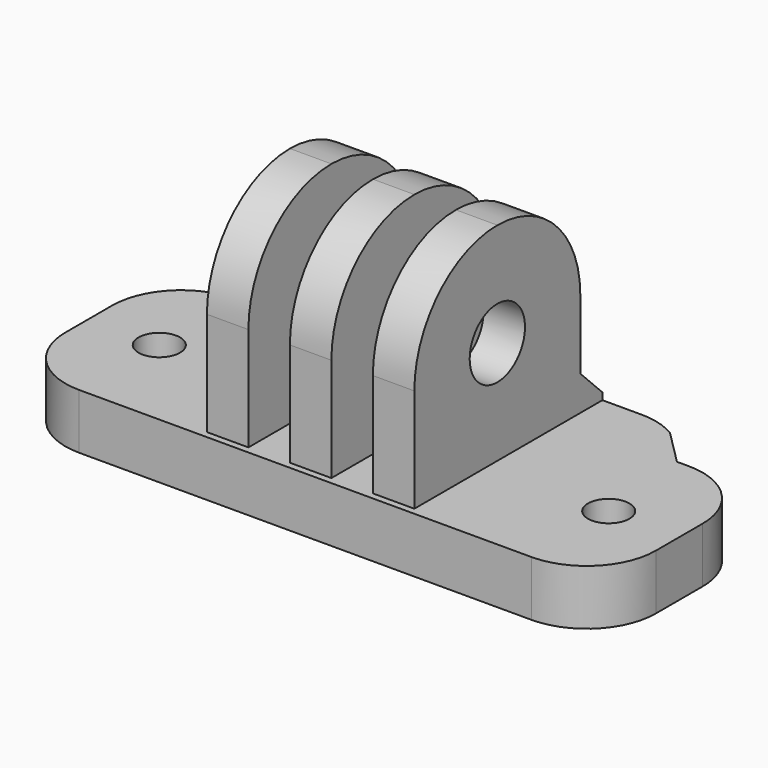
from build123d import *

# Parameters (mm, degrees)
F0_R         = 1.5
F0_W         = 3
F0_H         = 13.7437733207
F0_H_2       = 1.2562266793
F1_DEPTH     = 4
F2_DEPTH     = 19
F3_R         = 7.49999
F4_R         = 2.5
F5_DEPTH     = 28.851
F6_T1_DEPTH  = 4
F6_T6_DEPTH  = 3
F6_T11_DEPTH = 9.4292074699
F6_T18_DEPTH = 9.4292074699
F6_T25_DEPTH = 3
F6_T30_DEPTH = 9.4292074699
F6_T37_DEPTH = 9.4292074699
F6_T44_DEPTH = 3
F7_T1_DEPTH  = 17.2196709514
F7_T3_DEPTH  = 29


# Not quite as in the source:
# - a fillet or chamfer that OpenCascade refuses, or shapes differently, is made with other operations: its cross-section is extruded or revolved along the edge and cut away or added
# - a fillet or chamfer is up to 0.001 mm smaller than in the source, because OpenCascade refuses the exact size


with BuildPart() as f1:
    # F0 (on Top) → F1 (new body)
    with BuildSketch(Plane.XY):
        Polygon((-12.9930239742, 7.1134486855), (-21.35, 7.1134486855), (-21.35, -7.1134486855), (21.35, -7.1134486855), (21.35, 7.1134486855), (12.9930239742, 7.1134486855), (7.5, 7.1134486855), (7.5, -6.6303246352), (4.5, -6.6303246352), (4.5, 7.1134486855), (1.5, 7.1134486855), (1.5, -6.6303246352), (-1.5, -6.6303246352), (-1.5, 7.1134486855), (-4.5, 7.1134486855), (-4.5, -6.6303246352), (-7.5, -6.6303246352), (-7.5, 7.1134486855), align=None)
        with Locations((-16.25, 0)):
            Circle(F0_R, mode=Mode.SUBTRACT)
        with Locations((16.25, 0)):
            Circle(F0_R, mode=Mode.SUBTRACT)
        Polygon((-12.9930239742, 10.3696753648), (-12.9930239742, 7.1134486855), (-7.5, 7.1134486855), (-7.5, 8.3696753648), (-4.5, 8.3696753648), (-1.5, 8.3696753648), (1.5, 8.3696753648), (4.5, 8.3696753648), (7.5, 8.3696753648), (7.5, 7.1134486855), (12.9930239742, 7.1134486855), (12.9930239742, 10.3696753648), align=None)
        with Locations((-6, 0.2415620252)):
            Rectangle(F0_W, F0_H)
        with Locations((-6, 7.7415620252)):
            Rectangle(F0_W, F0_H_2)
        with Locations((-3, 7.7415620252)):
            Rectangle(F0_W, F0_H_2)
        Polygon((-1.5, 8.3696753648), (-1.5, 7.1134486855), (0, 7.1134486855), (1.5, 7.1134486855), (1.5, 8.3696753648), align=None)
        Polygon((0, 7.1134486855), (-1.5, 7.1134486855), (-1.5, -6.6303246352), (1.5, -6.6303246352), (1.5, 7.1134486855), align=None)
        with Locations((3, 7.7415620252)):
            Rectangle(F0_W, F0_H_2)
        with Locations((6, 0.2415620252)):
            Rectangle(F0_W, F0_H)
        with Locations((6, 7.7415620252)):
            Rectangle(F0_W, F0_H_2)
    extrude(amount=F1_DEPTH)

    # F0 (on Top) → F2 (join)
    with BuildSketch(Plane.XY):
        with Locations((-6, 0.2415620252)):
            Rectangle(F0_W, F0_H)
        with Locations((-6, 7.7415620252)):
            Rectangle(F0_W, F0_H_2)
        Polygon((-1.5, 8.3696753648), (-1.5, 7.1134486855), (0, 7.1134486855), (1.5, 7.1134486855), (1.5, 8.3696753648), align=None)
        Polygon((0, 7.1134486855), (-1.5, 7.1134486855), (-1.5, -6.6303246352), (1.5, -6.6303246352), (1.5, 7.1134486855), align=None)
        with Locations((6, 0.2415620252)):
            Rectangle(F0_W, F0_H)
        with Locations((6, 7.7415620252)):
            Rectangle(F0_W, F0_H_2)
    extrude(amount=F2_DEPTH)

    # F3 (radius 7.5 in the source; OpenCascade refuses exactly that, so slightly less here)
    f3_edges = [f1.edges().sort_by_distance(p)[0] for p in [
        (-6, -6.630325, 19),
        (0, -6.630325, 19),
        (6, -6.630325, 19),
        (6, 8.369675, 19),
        (0, 8.369675, 19),
        (-6, 8.369675, 19),
    ]]
    fillet(f3_edges, radius=F3_R)

    # F4 (on face) → F5 (cut, through all)
    with BuildSketch(Plane(origin=(-7.5, 0, 0), x_dir=(0, -1, 0), z_dir=(-1, 0, 0))):
        with Locations((-0.8696753648, 11.5)):
            Circle(F4_R)
    extrude(amount=-F5_DEPTH, mode=Mode.SUBTRACT)

    # F6: chamfer of 2.5 on 5 edges, made by hand

    # F6_s2 → F6_t1 (join)
    with BuildSketch(Plane.XY):
        Polygon((12.9930239742, 9.6134486855), (15.4930239742, 7.1134486855), (12.9930239742, 7.1134486855), align=None)
        Polygon((-15.4930239742, 7.1134486855), (-12.9930239742, 9.6134486855), (-12.9930239742, 7.1134486855), align=None)
    extrude(amount=F6_T1_DEPTH)


with BuildPart() as f6_tool4:
    # F6_s5 → F6_t6 (new body)
    with BuildSketch(Plane.YZ.offset(-7.5)):
        Polygon((8.3696753648, 6.5), (10.8696753648, 4), (8.3696753648, 4), align=None)
    extrude(amount=F6_T6_DEPTH)

    split(bisect_by=Plane.XZ.offset(-10.3696753648), keep=Keep.TOP)


with BuildPart() as f1_1:
    add(f1.part)

    # F6_t3: union F6_tool4
    add(f6_tool4.part)


with BuildPart() as f6_tool9:
    # F6_s10 → F6_t11 (new body)
    with BuildSketch(Plane.YZ.offset(-7.5)):
        Polygon((8.3696753648, 6.5), (10.8696753648, 4), (8.3696753648, 4), align=None)
    extrude(amount=F6_T11_DEPTH)

    split(bisect_by=Plane.XZ.offset(-10.3696753648), keep=Keep.TOP)

    split(bisect_by=Plane.YZ.offset(-1.5), keep=Keep.TOP)

    split(bisect_by=Plane.YZ.offset(1.5), keep=Keep.BOTTOM)


with BuildPart() as f1_2:
    add(f1_1.part)

    # F6_t8: union F6_tool9
    add(f6_tool9.part)


with BuildPart() as f6_tool16:
    # F6_s17 → F6_t18 (new body)
    with BuildSketch(Plane.YZ.offset(-7.9292074699)):
        Polygon((10.8696753648, 4), (8.3696753648, 6.5), (8.3696753648, 4), align=None)
    extrude(amount=F6_T18_DEPTH)

    split(bisect_by=Plane.YZ.offset(-7.5), keep=Keep.TOP)

    split(bisect_by=Plane.YZ.offset(-4.5), keep=Keep.BOTTOM)

    split(bisect_by=Plane.XZ.offset(-10.3696753648), keep=Keep.TOP)


with BuildPart() as f1_3:
    add(f1_2.part)

    # F6_t15: union F6_tool16
    add(f6_tool16.part)


with BuildPart() as f6_tool23:
    # F6_s24 → F6_t25 (new body)
    with BuildSketch(Plane.YZ.offset(-1.5)):
        Polygon((10.8696753648, 4), (8.3696753648, 6.5), (8.3696753648, 4), align=None)
    extrude(amount=F6_T25_DEPTH)

    split(bisect_by=Plane.XZ.offset(-10.3696753648), keep=Keep.TOP)


with BuildPart() as f1_4:
    add(f1_3.part)

    # F6_t22: union F6_tool23
    add(f6_tool23.part)


with BuildPart() as f6_tool28:
    # F6_s29 → F6_t30 (new body)
    with BuildSketch(Plane.YZ.offset(-1.5)):
        Polygon((10.8696753648, 4), (8.3696753648, 6.5), (8.3696753648, 4), align=None)
    extrude(amount=F6_T30_DEPTH)

    split(bisect_by=Plane.XZ.offset(-10.3696753648), keep=Keep.TOP)

    split(bisect_by=Plane.YZ.offset(4.5), keep=Keep.TOP)

    split(bisect_by=Plane.YZ.offset(7.5), keep=Keep.BOTTOM)


with BuildPart() as f1_5:
    add(f1_4.part)

    # F6_t27: union F6_tool28
    add(f6_tool28.part)


with BuildPart() as f6_tool35:
    # F6_s36 → F6_t37 (new body)
    with BuildSketch(Plane.YZ.offset(-1.9292074699)):
        Polygon((10.8696753648, 4), (8.3696753648, 6.5), (8.3696753648, 4), align=None)
    extrude(amount=F6_T37_DEPTH)

    split(bisect_by=Plane.XZ.offset(-10.3696753648), keep=Keep.TOP)

    split(bisect_by=Plane.YZ.offset(-1.5), keep=Keep.TOP)

    split(bisect_by=Plane.YZ.offset(1.5), keep=Keep.BOTTOM)


with BuildPart() as f1_6:
    add(f1_5.part)

    # F6_t34: union F6_tool35
    add(f6_tool35.part)


with BuildPart() as f6_tool42:
    # F6_s43 → F6_t44 (new body)
    with BuildSketch(Plane.YZ.offset(4.5)):
        Polygon((10.8696753648, 4), (8.3696753648, 6.5), (8.3696753648, 4), align=None)
    extrude(amount=F6_T44_DEPTH)

    split(bisect_by=Plane.XZ.offset(-10.3696753648), keep=Keep.TOP)


with BuildPart() as f1_7:
    add(f1_6.part)

    # F6_t41: union F6_tool42
    add(f6_tool42.part)

    # F7: fillet of radius 5 on 6 edges, made by hand

    # F7_s2 → F7_t1 (cut)
    with BuildSketch(Plane.XY.offset(-6.6098354757)):
        with BuildLine():
            ThreePointArc((10.3490897839, 10.3696753648), (11.7240685831, 10.1769025595), (12.9930239742, 9.6134486855))
            Line((12.9930239742, 9.6134486855), (12.9930239742, 10.3696753648))
            Line((12.9930239742, 10.3696753648), (10.3490897839, 10.3696753648))
        make_face()
        with BuildLine():
            ThreePointArc((-10.3490897839, 10.3696753648), (-11.7240685831, 10.1769025595), (-12.9930239742, 9.6134486855))
            Line((-12.9930239742, 9.6134486855), (-12.9930239742, 10.3696753648))
            Line((-12.9930239742, 10.3696753648), (-10.3490897839, 10.3696753648))
        make_face()
    extrude(amount=F7_T1_DEPTH, mode=Mode.SUBTRACT)

    # F7_s4 → F7_t3 (cut)
    with BuildSketch(Plane.XY.offset(-12.5)):
        with BuildLine():
            ThreePointArc((-21.35, 2.1134486855), (-19.8855339059, 5.6489825915), (-16.35, 7.1134486855))
            Line((-16.35, 7.1134486855), (-21.35, 7.1134486855))
            Line((-21.35, 7.1134486855), (-21.35, 2.1134486855))
        make_face()
        with BuildLine():
            ThreePointArc((-16.35, -7.1134486855), (-19.8855339059, -5.6489825915), (-21.35, -2.1134486855))
            Line((-21.35, -2.1134486855), (-21.35, -7.1134486855))
            Line((-21.35, -7.1134486855), (-16.35, -7.1134486855))
        make_face()
        with BuildLine():
            ThreePointArc((21.35, -2.1134486855), (19.8855339059, -5.6489825915), (16.35, -7.1134486855))
            Line((16.35, -7.1134486855), (21.35, -7.1134486855))
            Line((21.35, -7.1134486855), (21.35, -2.1134486855))
        make_face()
        with BuildLine():
            ThreePointArc((16.35, 7.1134486855), (19.8855339059, 5.6489825915), (21.35, 2.1134486855))
            Line((21.35, 2.1134486855), (21.35, 7.1134486855))
            Line((21.35, 7.1134486855), (16.35, 7.1134486855))
        make_face()
    extrude(amount=F7_T3_DEPTH, mode=Mode.SUBTRACT)


solid = f1_7.part
